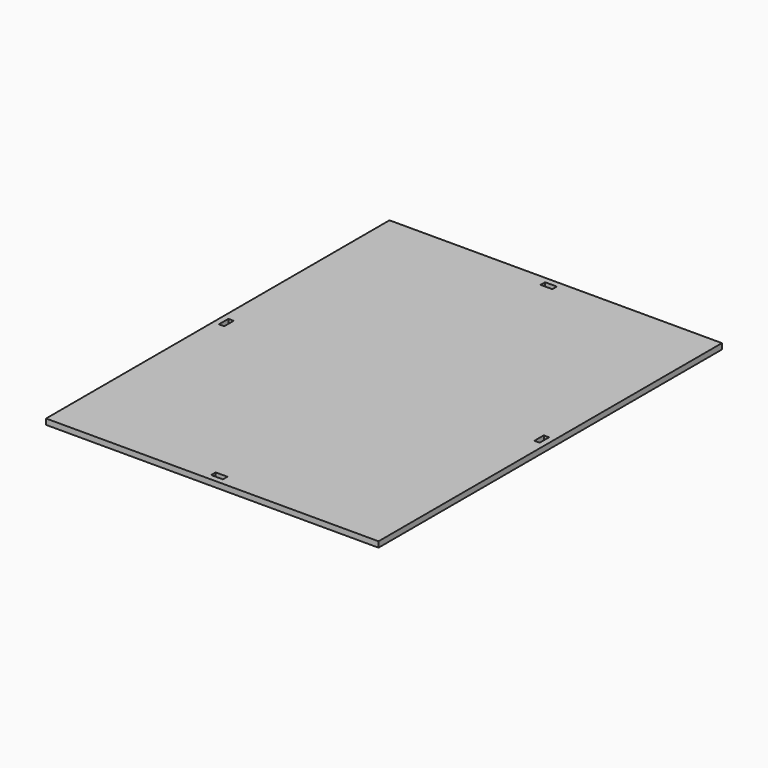
from build123d import *

# Parameters (mm, degrees)
F1_DEPTH = 4.8
F2_DEPTH = 4.8


# Not quite as in the source:
# - a feature names something its author has since deleted; it is built from what else it names


with BuildPart() as f1:
    # F0 (on Top) → F1 (new body)
    with BuildSketch(Plane.XY):
        Polygon((140.7586729476, 255.9633882557), (9.5784879476, 255.9633882557), (9.5784879476, 251.1633882557), (4.5784879476, 251.1633882557), (4.5784879476, 78.6871632557), (4.5784879476, -93.7890617443), (9.5784879476, -93.7890617443), (9.5784879476, -98.5890617443), (140.7586729476, -98.5890617443), (140.7586729476, 73.6871632557), (136.2586729476, 73.6871632557), (136.2586729476, 78.6871632557), (136.2586729476, 83.6871632557), (140.7586729476, 83.6871632557), align=None)
        Polygon((-0.4215120524, 255.9633882557), (-131.6016970524, 255.9633882557), (-131.6016970524, 83.6871632557), (-127.1016970524, 83.6871632557), (-127.1016970524, 78.6871632557), (-127.1016970524, 73.6871632557), (-131.6016970524, 73.6871632557), (-131.6016970524, -98.5890617443), (-0.4215120524, -98.5890617443), (-0.4215120524, -93.7890617443), (4.5784879476, -93.7890617443), (4.5784879476, 78.6871632557), (4.5784879476, 251.1633882557), (-0.4215120524, 251.1633882557), align=None)
        Polygon((-131.6016970524, 83.6871632557), (-131.6016970524, 255.9633882557), (-0.4215120524, 255.9633882557), (9.5784879476, 255.9633882557), (140.7586729476, 255.9633882557), (140.7586729476, 260.9633888568), (-136.6016970524, 260.9633888568), (-136.6016970524, -103.5890617443), (-131.6016970524, -103.5890617443), (-131.6016970524, -98.5890617443), (-131.6016970524, 73.6871632557), (-131.6016970524, 78.6871632557), align=None)
    extrude(amount=F1_DEPTH)

    # F0 (on Top) → F2 (join)
    with BuildSketch(Plane.XY):
        Polygon((-131.6016970524, 83.6871632557), (-131.6016970524, 255.9633882557), (-0.4215120524, 255.9633882557), (9.5784879476, 255.9633882557), (140.7586729476, 255.9633882557), (140.7586729476, 260.9633888568), (-136.6016970524, 260.9633888568), (-136.6016970524, -103.5890617443), (-131.6016970524, -103.5890617443), (-131.6016970524, -98.5890617443), (-131.6016970524, 73.6871632557), (-131.6016970524, 78.6871632557), align=None)
        Polygon((140.7586729476, 260.9633888568), (140.7586729476, 255.9633882557), (140.7586729476, 83.6871632557), (140.7586729476, 78.6871632557), (140.7586729476, 73.6871632557), (140.7586729476, -98.5890617443), (9.5784879476, -98.5890617443), (-0.4215120524, -98.5890617443), (-131.6016970524, -98.5890617443), (-131.6016970524, -103.5890617443), (145.7586729476, -103.5890617443), (145.7586729476, 260.9633888568), align=None)
    extrude(amount=F2_DEPTH)


solid = f1.part
